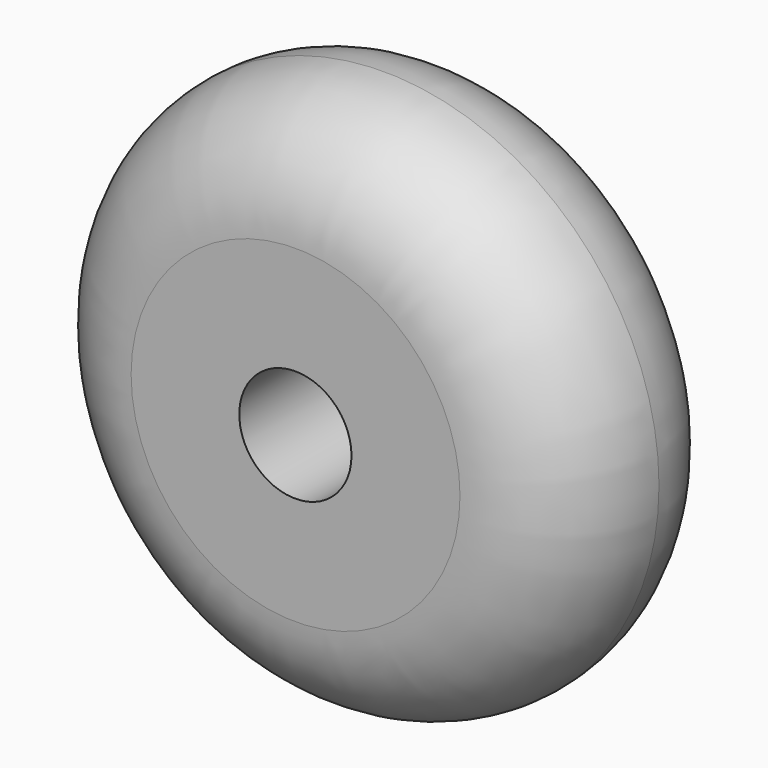
from build123d import *

# Parameters (mm, degrees)
F0_R     = 12.6376963258
F1_DEPTH = 10.16
F2_R     = 5.07999
F3_R     = 2.5783631355
F4_DEPTH = 25.4


# Not quite as in the source:
# - a fillet or chamfer is up to 0.001 mm smaller than in the source, because OpenCascade refuses the exact size


with BuildPart() as f1:
    # F0 (on Front) → F1 (new body)
    with BuildSketch(Plane.XZ):
        with Locations((-57.7037265382, 0)):
            Circle(F0_R)
    extrude(amount=F1_DEPTH)

    # F2 (radius 5.08 in the source; OpenCascade refuses exactly that, so slightly less here)
    f2_edges = [f1.edges().sort_by_distance(p)[0] for p in [
        (-70.341423, 0, 0),
        (-70.341423, -10.16, 0),
    ]]
    fillet(f2_edges, radius=F2_R)

    # F3 (on Front) → F4 (cut)
    with BuildSketch(Plane.XZ):
        with Locations((-57.7121302485, 0)):
            Circle(F3_R)
    extrude(amount=F4_DEPTH, mode=Mode.SUBTRACT)


solid = f1.part
